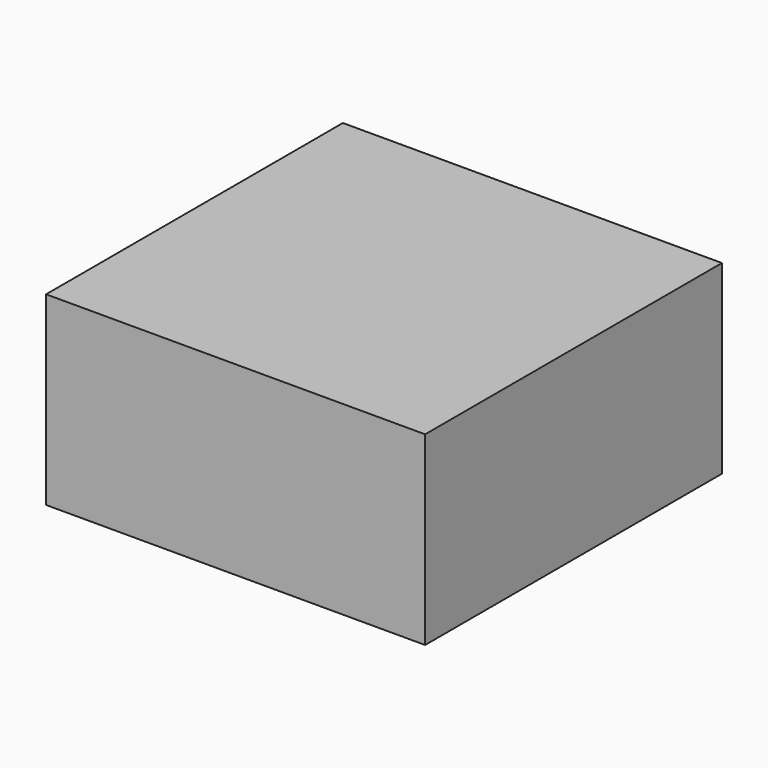
from build123d import *

# Parameters (mm, degrees)
F1_W     = 5969
F1_H     = 5842
F2_DEPTH = 2921


# Not quite as in the source:
# - a variable given as a bare number and used for a length is read in inches; the dataset says mm whatever the document's units were


with BuildPart() as f2:
    # F1 (on Top) → F2 (new body)
    with BuildSketch(Plane.XY):
        Rectangle(F1_W, F1_H)
    extrude(amount=F2_DEPTH)


solid = f2.part
